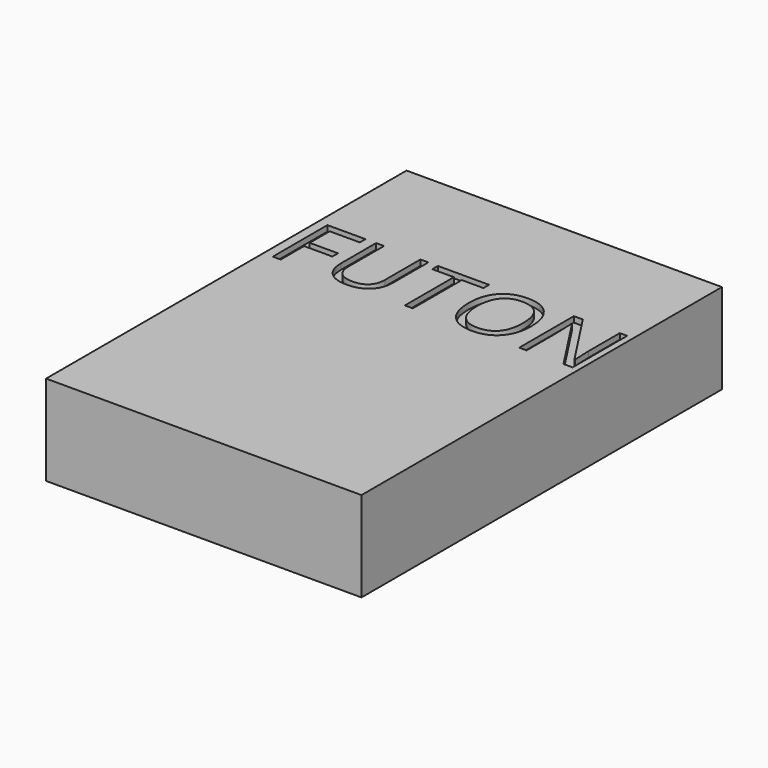
from build123d import *

# Parameters (mm, degrees)
F0_W         = 1400.175
F0_H         = 2000.25
F1_DEPTH     = 200.025
F2_TEXT_SIZE = 424.7177591355
F3_DEPTH     = 25.4


# Not quite as in the source:
# - Text() gives the source's letters only with a copy of the font that has no kerning and outlines rounded to 1/6400 em; it was checked with that copy


with BuildPart() as f1:
    # F0 (on Top) → F1 (new body, symmetric)
    with BuildSketch(Plane.XY):
        Rectangle(F0_W, F0_H)
    extrude(amount=F1_DEPTH, both=True)

    # F2 (on face) → F3 (cut)
    with BuildSketch(Plane.XY.offset(200.025)):
        with Locations((-700.0875, 205.7735276119)):
            Text('FUTON', F2_TEXT_SIZE, font='Open Sans', text_align=(TextAlign.LEFT, TextAlign.BOTTOM))
    extrude(amount=-F3_DEPTH, mode=Mode.SUBTRACT)


solid = f1.part
